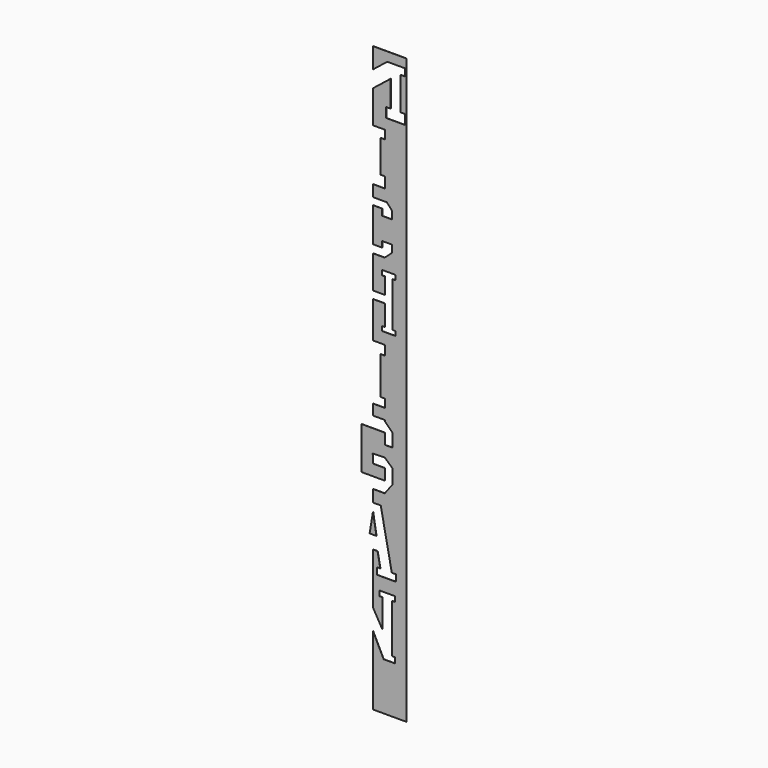
from build123d import *

# Parameters (mm, degrees)
F0_W     = 5.2482880054
F0_H     = 4.9810466543
F1_DEPTH = 0.0762


# Not quite as in the source:
# - a feature names something its author has since deleted; it is built from what else it names


with BuildPart() as f1:
    # F0 (on Front) → F1 (new body)
    with BuildSketch(Plane.XZ):
        Polygon((-35.1963832856, 79.4969911185), (-50.193608411, 79.4969911185), (-50.193608411, 70.3488993556), (-43.8295094164, 75.4326850121), (-35.9808335364, 75.4326850121), (-35.9808335364, 72.2227817215), (-37.8685602848, 72.2227817215), (-37.8685602848, 57.4692988183), (-35.9808335364, 57.4692988183), (-35.9808335364, 53.1461095161), (-44.2987100306, 53.1461095161), (-44.2987100306, 57.4692988183), (-42.2831444735, 57.4692988183), (-42.2831444735, 69.2738860086), (-50.193608411, 62.954829197), (-50.193608411, 48.3592389848), (-44.9453204056, 48.3592389848), (-44.9453204056, 44.5231835829), (-46.7674447154, 44.5231835829), (-46.7674447154, 30.0220460158), (-44.9453204056, 30.0220460158), (-44.9453204056, 25.2169134009), (-50.193608411, 25.2169134009), (-50.193608411, 20.1037506657), (-44.0339450055, 20.1037506657), (-41.6973850482, 17.5189805853), (-41.6973850482, 14.0874953759), (-46.0979307142, 14.0874953759), (-46.0979307142, 16.9323027027), (-50.193608411, 16.9323027027), (-50.193608411, 1.5689273412), (-46.0979307142, 1.5689273412), (-46.0979307142, 4.1895659023), (-41.6973850482, 4.1895659023), (-41.6973850482, 0.9874830587), (-44.9919385552, -1.9907012912), (-50.193608411, -1.9907012912), (-50.193608411, -16.6316394584), (-44.9453204056, -16.6316394584), (-44.9453204056, -9.343899268), (-46.1852711141, -9.343899268), (-46.1852711141, -7.1931303074), (-44.9453204056, -7.1931303074), (-41.4369731104, -7.1931303074), (-40.111375595, -7.1931303074), (-40.111375595, -9.343899268), (-41.4369731104, -9.343899268), (-41.4369731104, -29.2911320519), (-40.111375595, -29.2911320519), (-40.111375595, -31.2461041507), (-41.4369731104, -31.2461041507), (-44.9453204056, -31.2461041507), (-46.1852711141, -31.2461041507), (-46.1852711141, -29.2911320519), (-44.9453204056, -29.2911320519), (-44.9453204056, -19.9807869131), (-50.193608411, -19.9807869131), (-50.193608411, -36.2698242769), (-44.9453204056, -36.2698242769), (-44.9453204056, -40.5323778866), (-46.7674447154, -40.5323778866), (-46.7674447154, -57.3903505305), (-44.9453204056, -57.3903505305), (-44.9453204056, -61.0807400528), (-50.193608411, -61.0807400528), (-50.193608411, -65.8248991014), (-44.9453204056, -65.8248991014), (-44.9453204056, -66.3401821199), (-41.4369731104, -69.7753881654), (-41.4369731104, -75.6152342194), (-44.9453204056, -75.6152342194), (-44.9453204056, -70.8059457557), (-50.193608411, -70.8059457557), (-50.193608411, -73.4616260623), (-50.193608411, -80.7633897693), (-44.9453204056, -80.5831793362), (-41.5694830255, -83.6879705381), (-41.5694830255, -90.214866248), (-44.9453204056, -94.6806298838), (-50.193608411, -94.6806298838), (-50.193608411, -100.0432713063), (-46.7460826389, -100.0432713063), (-41.7978071284, -124.8997201194), (-40.0056464088, -124.8997201194), (-40.0056464088, -127.8638071794), (-41.2077341248, -127.8638071794), (-46.3596858381, -127.8638071794), (-48.4354351813, -127.8397336649), (-48.4354351813, -124.8997201194), (-46.9281419303, -124.8997201194), (-48.1628723165, -118.4614948803), (-50.193608411, -118.4614948803), (-50.193608411, -141.3308172114), (-46.009728736, -148.5575184684), (-46.009728736, -135.918805119), (-47.3438533436, -135.918805119), (-47.3438533436, -135.2590725668), (-47.3438533436, -133.6447787085), (-46.009728736, -133.6447787085), (-41.7978071284, -133.6447787085), (-40.4277944904, -133.6447787085), (-40.4089242338, -135.918805119), (-41.7978071284, -135.918805119), (-41.7978071284, -157.6631183666), (-40.4089242338, -157.6631183666), (-40.4089242338, -160.1064702757), (-41.7978071284, -160.1064702757), (-45.4491030418, -160.1064702757), (-50.193608411, -150.5596009381), (-50.193608411, -181.4232210127), (-35.1963832856, -181.4232210127), (-35.1963832856, -73.4616260623), (-35.1963832856, 72.2227817215), (-35.1963832856, 75.4326850121), align=None)
        with Locations((-47.5694644083, -87.2090599023)):
            Rectangle(F0_W, F0_H)
        Polygon((-55.4418964164, -89.6995832295), (-50.193608411, -89.6995832295), (-50.193608411, -84.7185365752), (-50.3292563299, -80.7680475111), (-50.193608411, -80.7633897693), (-50.193608411, -73.4616260623), (-50.193608411, -70.8059457557), (-55.4418964164, -70.8059457557), align=None)
    extrude(amount=F1_DEPTH)


with BuildPart() as f1b:
    # F0 (on Front) → F1, piece 2 (new body)
    with BuildSketch(Plane.XZ):
        Polygon((-51.709150179, -112.6655470911), (-50.193608411, -112.6655470911), (-50.193608411, -103.5208382904), align=None)
        Polygon((-50.193608411, -103.5208382904), (-50.193608411, -112.6655470911), (-48.6780666431, -112.6655470911), align=None)
    extrude(amount=F1_DEPTH)


solid = Compound([f1.part, f1b.part])
